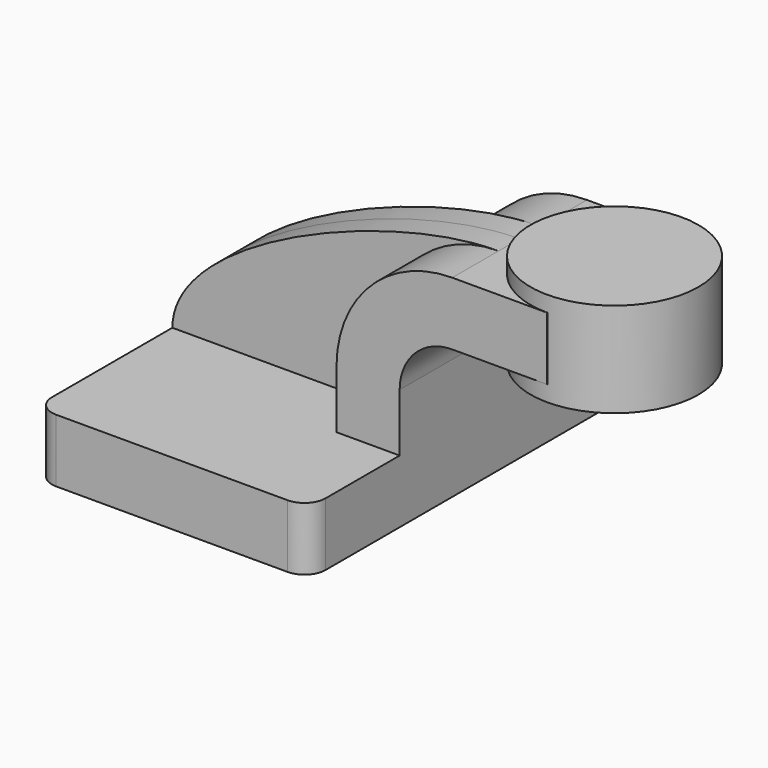
from build123d import *

# Parameters (mm, degrees)
F1_DEPTH = 59.69
F2_DEPTH = 25.4
F4_DEPTH = 7.9375
F6_R     = 6.35


# Not quite as in the source:
# - a feature of the source that left no trace in its solid (it failed there, or was rolled back) is left out


with BuildPart() as f1:
    # F0 (on Front) → F1 (new body, symmetric)
    with BuildSketch(Plane.XZ):
        Polygon((22.225, 9.525), (-41.275, 9.525), (-41.275, -9.525), (41.275, -9.525), (41.275, 9.525), align=None)
    extrude(amount=F1_DEPTH, both=True)

    # F0 (on Front) → F2 (join, symmetric)
    with BuildSketch(Plane.XZ):
        with BuildLine():
            Line((22.225, 27.0002), (22.225, 9.525))
            Line((22.225, 9.525), (41.275, 9.525))
            Line((41.275, 9.525), (41.275, 27.0002))
            ThreePointArc((41.275, 27.0002), (45.9246798487, 38.2255201513), (57.15, 42.8752))
            Line((57.15, 42.8752), (60.325, 42.8752))
            Line((60.325, 42.8752), (60.325, 61.9252))
            Line((60.325, 61.9252), (57.15, 61.9252))
            ThreePointArc((57.15, 61.9252), (32.4542956671, 51.6959043329), (22.225, 27.0002))
        make_face()
        Polygon((85.7749970019, 61.9252), (60.325, 61.9252), (60.325, 42.8752), (85.7749970019, 42.8752), (85.7749970019, 46.5751625597), align=None)
    extrude(amount=F2_DEPTH, both=True)

    # F0 (on Front) → F4 (join, symmetric)
    with BuildSketch(Plane.XZ):
        with BuildLine():
            add(Edge.make_bspline(
                [(-41.275, 9.525), (-41.1301143467, 35.7692055404), (24.3351403624, 62.0320998132), (57.15, 61.9252)],
                knots=[0, 0, 0, 0, 111.5045361635, 111.5045361635, 111.5045361635, 111.5045361635], degree=3))
            Line((-41.275, 9.525), (22.225, 9.525))
            Line((22.225, 9.525), (22.225, 27.0002))
            ThreePointArc((22.225, 27.0002), (32.4542956671, 51.6959043329), (57.15, 61.9252))
        make_face()
    extrude(amount=F4_DEPTH, both=True)

    # F0 (on Front) → F5 (revolve)
    with BuildSketch(Plane.XZ):
        Polygon((85.7749970019, 66.675), (85.7749970019, 61.9252), (85.7749970019, 46.5751625597), (85.7749970019, 42.8752), (85.7749970019, 38.1), (111.125, 38.1), (111.125, 66.675), align=None)
    revolve(axis=Axis((85.7749970019, 0, 56.6250812799), (0, 0, 1)))

    # F6
    f6_edges = [f1.edges().sort_by_distance(p)[0] for p in [
        (41.275, -59.69, 0),
        (-41.275, -59.69, 0),
        (-41.275, 59.69, 0),
        (41.275, 59.69, 0),
    ]]
    fillet(f6_edges, radius=F6_R)


solid = f1.part
